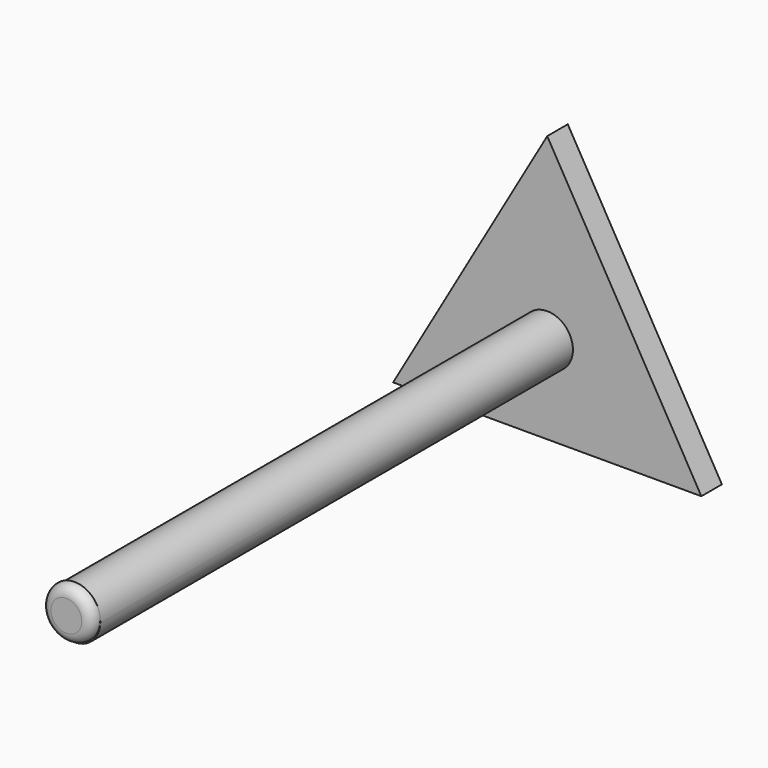
from build123d import *

# Parameters (mm, degrees)
F1_DEPTH = 12.7
F2_R     = 12.7
F3_DEPTH = 304.8
F4_R     = 12.7
F5_DEPTH = 5.08
F6_R     = 5.07999


# Not quite as in the source:
# - a fillet or chamfer is up to 0.001 mm smaller than in the source, because OpenCascade refuses the exact size


with BuildPart() as f1:
    # F0 (on Front) → F1 (new body)
    with BuildSketch(Plane.XZ):
        Polygon((-76.2, -43.9940905122), (76.2, -43.9940905122), (0, 87.9881810245), align=None)
    extrude(amount=F1_DEPTH)

    # F2 (on Front) → F3 (join)
    with BuildSketch(Plane.XZ):
        with Locations((0, -0.8957827414)):
            Circle(F2_R)
    extrude(amount=F3_DEPTH)

    # F4 (on face) → F5 (join)
    with BuildSketch(Plane.XZ.offset(304.8)):
        Circle(F4_R)
    extrude(amount=F5_DEPTH)

    # F6 (radius 5.08 in the source; OpenCascade refuses exactly that, so slightly less here)
    f6_edges = [f1.edges().sort_by_distance(p)[0] for p in [
        (-12.7, -309.88, 0),
    ]]
    fillet(f6_edges, radius=F6_R)


solid = f1.part
